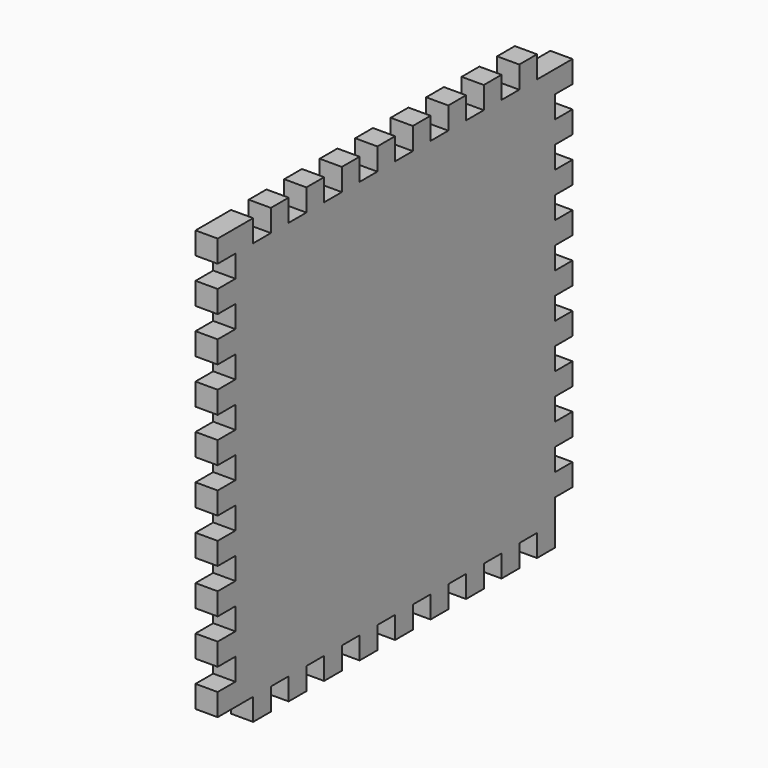
from build123d import *

# Parameters (mm, degrees)
F1_DEPTH = 6.35


# Not quite as in the source:
# - a feature names something its author has since deleted; it is built from what else it names


with BuildPart() as f1:
    # F0 (on Right) → F1 (new body)
    with BuildSketch(Plane.YZ):
        Polygon((12.7, 127), (6.35, 127), (0, 127), (0, 120.65), (6.35, 120.65), (6.35, 114.3), (0, 114.3), (0, 107.95), (6.35, 107.95), (6.35, 101.6), (0, 101.6), (0, 95.25), (6.35, 95.25), (6.35, 88.9), (0, 88.9), (0, 82.55), (6.35, 82.55), (6.35, 76.2), (0, 76.2), (0, 69.85), (6.35, 69.85), (6.35, 63.5), (0, 63.5), (0, 57.15), (6.35, 57.15), (6.35, 50.8), (0, 50.8), (0, 44.45), (6.35, 44.45), (6.35, 38.1), (0, 38.1), (0, 31.75), (6.35, 31.75), (6.35, 25.4), (0, 25.4), (0, 19.05), (6.35, 19.05), (6.35, 12.7), (0, 12.7), (0, 6.35), (6.35, 6.35), (12.7, 6.35), (12.7, 0), (19.05, 0), (19.05, 6.35), (25.4, 6.35), (25.4, 0), (31.75, 0), (31.75, 6.35), (38.1, 6.35), (38.1, 0), (44.45, 0), (44.45, 6.35), (50.8, 6.35), (50.8, 0), (57.15, 0), (57.15, 6.35), (63.5, 6.35), (63.5, 0), (69.85, 0), (69.85, 6.35), (76.2, 6.35), (76.2, 0), (82.55, 0), (82.55, 6.35), (88.9, 6.35), (88.9, 0), (95.25, 0), (95.25, 6.35), (101.6, 6.35), (101.6, 0), (107.95, 0), (107.95, 6.35), (114.3, 6.35), (114.3, 0), (120.65, 0), (120.65, 6.35), (120.65, 12.7), (127, 12.7), (127, 19.05), (120.65, 19.05), (120.65, 25.4), (127, 25.4), (127, 31.75), (120.65, 31.75), (120.65, 38.1), (127, 38.1), (127, 44.45), (120.65, 44.45), (120.65, 50.8), (127, 50.8), (127, 57.15), (120.65, 57.15), (120.65, 63.5), (127, 63.5), (127, 69.85), (120.65, 69.85), (120.65, 76.2), (127, 76.2), (127, 82.55), (120.65, 82.55), (120.65, 88.9), (127, 88.9), (127, 95.25), (120.65, 95.25), (120.65, 101.6), (127, 101.6), (127, 107.95), (120.65, 107.95), (120.65, 114.3), (127, 114.3), (127, 120.65), (120.65, 120.65), (114.3, 120.65), (114.3, 127), (107.95, 127), (107.95, 120.65), (101.6, 120.65), (101.6, 127), (95.25, 127), (95.25, 120.65), (88.9, 120.65), (88.9, 127), (82.55, 127), (82.55, 120.65), (76.2, 120.65), (76.2, 127), (69.85, 127), (69.85, 120.65), (63.5, 120.65), (63.5, 127), (57.15, 127), (57.15, 120.65), (50.8, 120.65), (50.8, 127), (44.45, 127), (44.45, 120.65), (38.1, 120.65), (38.1, 127), (31.75, 127), (31.75, 120.65), (25.4, 120.65), (25.4, 127), (19.05, 127), (19.05, 120.65), (12.7, 120.65), align=None)
    extrude(amount=F1_DEPTH)


solid = f1.part
